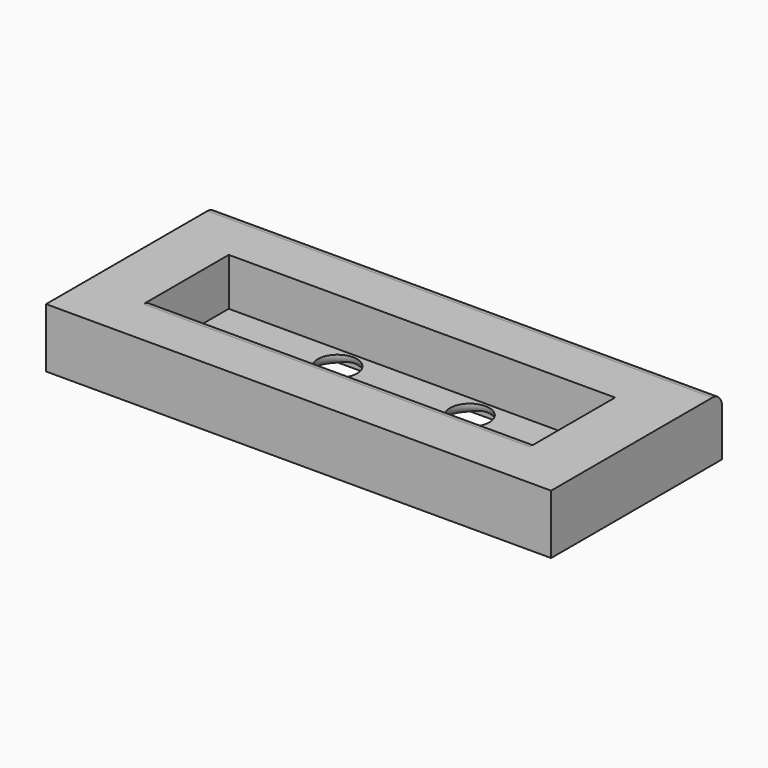
from build123d import *

# Parameters (mm, degrees)
F0_W        = 216.1347998985
F0_H        = 91.3698120594
F0_W_2      = 165.3347998985
F0_H_2      = 40.5698120594
F1_DEPTH    = 25.4
F0_R        = 8.376235911
F2_DEPTH    = 5.08
F3_T1_DEPTH = 190.7347998985
F3_T3_DEPTH = 65.9698120594
F3_2_F1_R   = 5.08
F3_2_F2_R   = 5.08


# Not quite as in the source:
# - a fillet or chamfer that OpenCascade refuses, or shapes differently, is made with other operations: its cross-section is extruded or revolved along the edge and cut away or added


with BuildPart() as f1:
    # F0 (on Top) → F1 (new body)
    with BuildSketch(Plane.XY):
        Rectangle(F0_W, F0_H)
        Rectangle(F0_W_2, F0_H_2, mode=Mode.SUBTRACT)
    extrude(amount=F1_DEPTH)

    # F3#2: fillet of radius 5.08 on 2 edges, made by hand

    # F3_2_f1
    f3_2_f1_edges = [f1.edges().sort_by_distance(p)[0] for p in [
        (0, 45.6849060297, 25.4),
    ]]
    fillet(f3_2_f1_edges, radius=F3_2_F1_R)

    # F3_2_f2
    f3_2_f2_edges = [f1.edges().sort_by_distance(p)[0] for p in [
        (0, -20.2849060297, 25.4),
    ]]
    fillet(f3_2_f2_edges, radius=F3_2_F2_R)


with BuildPart() as f2:
    # F0 (on Top) → F2 (new body)
    with BuildSketch(Plane.XY):
        Rectangle(F0_W_2, F0_H_2)
        with Locations((-28.30969356, -10.4768136516)):
            Circle(F0_R, mode=Mode.SUBTRACT)
        with Locations((28.30969356, -10.4768136516)):
            Circle(F0_R, mode=Mode.SUBTRACT)
        with Locations((-28.30969356, 10.4768136516)):
            Circle(F0_R, mode=Mode.SUBTRACT)
        with Locations((28.30969356, 10.4768136516)):
            Circle(F0_R, mode=Mode.SUBTRACT)
    extrude(amount=F2_DEPTH)

    # F3: fillet of radius 5.08 on 8 edges, made by hand

    # F3_s2 → F3_t1 (cut)
    with BuildSketch(Plane.YZ.offset(-95.3673999493)):
        with BuildLine():
            ThreePointArc((-20.2849060297, 5.08), (-18.7970084781, 1.4878975516), (-15.2049060297, 0))
            Line((-15.2049060297, 0), (-20.2849060297, 0))
            Line((-20.2849060297, 0), (-20.2849060297, 5.08))
        make_face()
        with BuildLine():
            ThreePointArc((20.2849060297, 5.08), (18.7970084781, 1.4878975516), (15.2049060297, 0))
            Line((15.2049060297, 0), (20.2849060297, 0))
            Line((20.2849060297, 0), (20.2849060297, 5.08))
        make_face()
    extrude(amount=F3_T1_DEPTH, mode=Mode.SUBTRACT)

    # F3_s4 → F3_t3 (cut)
    with BuildSketch(Plane.XZ.offset(-32.9849060297)):
        with BuildLine():
            ThreePointArc((82.6673999493, 5.08), (81.1795023977, 1.4878975516), (77.5873999493, 0))
            Line((77.5873999493, 0), (82.6673999493, 0))
            Line((82.6673999493, 0), (82.6673999493, 5.08))
        make_face()
        with BuildLine():
            ThreePointArc((-82.6673999493, 5.08), (-81.1795023977, 1.4878975516), (-77.5873999493, 0))
            Line((-77.5873999493, 0), (-82.6673999493, 0))
            Line((-82.6673999493, 0), (-82.6673999493, 5.08))
        make_face()
    extrude(amount=F3_T3_DEPTH, mode=Mode.SUBTRACT)

    # F3_s5 → F3_t6 (revolve, cut)
    with BuildSketch(Plane.XZ.offset(10.4768136516)):
        with BuildLine():
            ThreePointArc((-19.933457649, 5.08), (-18.4455600975, 1.4878975516), (-14.853457649, 0))
            Line((-14.853457649, 0), (-19.933457649, 0))
            Line((-19.933457649, 0), (-19.933457649, 5.08))
        make_face()
    revolve(axis=Axis((-28.30969356, -10.4768136516, 0), (0, 0, 1)), mode=Mode.SUBTRACT)

    # F3_s7 → F3_t8 (revolve, cut)
    with BuildSketch(Plane.XZ.offset(10.4768136516)):
        with BuildLine():
            ThreePointArc((36.685929471, 5.08), (38.1738270226, 1.4878975516), (41.765929471, 0))
            Line((41.765929471, 0), (36.685929471, 0))
            Line((36.685929471, 0), (36.685929471, 5.08))
        make_face()
    revolve(axis=Axis((28.30969356, -10.4768136516, 0), (0, 0, 1)), mode=Mode.SUBTRACT)

    # F3_s9 → F3_t10 (revolve, cut)
    with BuildSketch(Plane.XZ.offset(-10.4768136516)):
        with BuildLine():
            ThreePointArc((-19.933457649, 5.08), (-18.4455600975, 1.4878975516), (-14.853457649, 0))
            Line((-14.853457649, 0), (-19.933457649, 0))
            Line((-19.933457649, 0), (-19.933457649, 5.08))
        make_face()
    revolve(axis=Axis((-28.30969356, 10.4768136516, 0), (0, 0, 1)), mode=Mode.SUBTRACT)

    # F3_s11 → F3_t12 (revolve, cut)
    with BuildSketch(Plane.XZ.offset(-10.4768136516)):
        with BuildLine():
            ThreePointArc((36.685929471, 5.08), (38.1738270226, 1.4878975516), (41.765929471, 0))
            Line((41.765929471, 0), (36.685929471, 0))
            Line((36.685929471, 0), (36.685929471, 5.08))
        make_face()
    revolve(axis=Axis((28.30969356, 10.4768136516, 0), (0, 0, 1)), mode=Mode.SUBTRACT)


solid = Compound([f1.part, f2.part])
